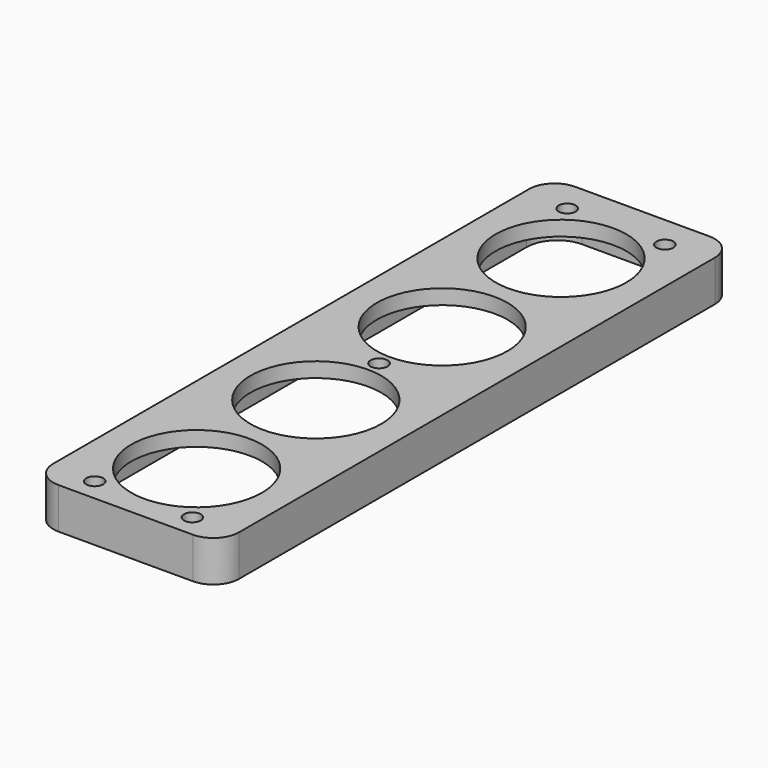
from build123d import *

# Parameters (mm, degrees)
F1_START      = 3.1
F0_W          = 32
F0_H          = 122
F0_R          = 1.65
F0_R_2        = 1.25
F0_R_3        = 12.75
F1_DEPTH      = 2.9
F2_START      = 3
F0_R_4        = 2
F0_R_5        = 1
F2_DEPTH      = 2
F3_DEPTH      = 25
F3_DEPTH_BACK = 39.8
F0_W_2        = 36.2426135689
F0_H_2        = 125.9943731129
F4_DEPTH      = 2
F4_DEPTH_BACK = 6
F5_R          = 6
F6_R          = 5


# Not quite as in the source:
# - a feature names something its author has since deleted; it is built from what else it names


with BuildPart() as f1:
    # F0 (on Top) → F1 (new body)
    with BuildSketch(Plane.XY.offset(F1_START)):
        with Locations((0, 0.9860133167)):
            Rectangle(F0_W, F0_H)
        with Locations((-9.525, -57.4329458177)):
            Circle(F0_R, mode=Mode.SUBTRACT)
        with Locations((-9.525, -30.4671674967)):
            Circle(F0_R_2, mode=Mode.SUBTRACT)
        with Locations((0, -44.4789328166)):
            Circle(F0_R_3, mode=Mode.SUBTRACT)
        with Locations((-9.525, 0)):
            Circle(F0_R_2, mode=Mode.SUBTRACT)
        with Locations((0, -15.4157546586)):
            Circle(F0_R_3, mode=Mode.SUBTRACT)
        Circle(F0_R, mode=Mode.SUBTRACT)
        with Locations((9.525, -57.4329458177)):
            Circle(F0_R, mode=Mode.SUBTRACT)
        with Locations((9.525, -30.4671674967)):
            Circle(F0_R_2, mode=Mode.SUBTRACT)
        with Locations((9.525, 0)):
            Circle(F0_R_2, mode=Mode.SUBTRACT)
        with Locations((-9.525, 29.1974432766)):
            Circle(F0_R_2, mode=Mode.SUBTRACT)
        with Locations((0, 15.3948861798)):
            Circle(F0_R_3, mode=Mode.SUBTRACT)
        with Locations((-9.525, 57.7905103564)):
            Circle(F0_R, mode=Mode.SUBTRACT)
        with Locations((0, 44.3624239764)):
            Circle(F0_R_3, mode=Mode.SUBTRACT)
        with Locations((9.525, 29.1974432766)):
            Circle(F0_R_2, mode=Mode.SUBTRACT)
        with Locations((9.525, 57.7905103564)):
            Circle(F0_R, mode=Mode.SUBTRACT)
        with Locations((9.525, 0)):
            Circle(F0_R_2)
        with Locations((-9.525, 0)):
            Circle(F0_R_2)
        with Locations((9.525, 29.1974432766)):
            Circle(F0_R_2)
        with Locations((-9.525, 29.1974432766)):
            Circle(F0_R_2)
        with Locations((9.525, -30.4671674967)):
            Circle(F0_R_2)
        with Locations((-9.525, -30.4671674967)):
            Circle(F0_R_2)
        with Locations((9.525, -57.4329458177)):
            Circle(F0_R)
        with Locations((-9.525, -57.4329458177)):
            Circle(F0_R)
        Circle(F0_R)
        with Locations((9.525, 57.7905103564)):
            Circle(F0_R)
        with Locations((-9.525, 57.7905103564)):
            Circle(F0_R)
    extrude(amount=F1_DEPTH)

    # F0 (on Top) → F2 (cut)
    with BuildSketch(Plane.XY.offset(F2_START)):
        with Locations((0, 44.3624239764)):
            Circle(F0_R_3)
        with Locations((-9.525, 44.3624239764)):
            Circle(F0_R_4, mode=Mode.SUBTRACT)
        with Locations((9.525, 44.3624239764)):
            Circle(F0_R_4, mode=Mode.SUBTRACT)
        with Locations((0, 15.3948861798)):
            Circle(F0_R_3)
        with Locations((-9.525, 15.3948861798)):
            Circle(F0_R_4, mode=Mode.SUBTRACT)
        with Locations((9.525, 15.3948861798)):
            Circle(F0_R_4, mode=Mode.SUBTRACT)
        with Locations((0, -15.4157546586)):
            Circle(F0_R_3)
        with Locations((-9.525, -15.4157546586)):
            Circle(F0_R_4, mode=Mode.SUBTRACT)
        with Locations((9.525, -15.4157546586)):
            Circle(F0_R_4, mode=Mode.SUBTRACT)
        with Locations((0, -44.4789328166)):
            Circle(F0_R_3)
        with Locations((-9.525, -44.4789328166)):
            Circle(F0_R_4, mode=Mode.SUBTRACT)
        with Locations((9.525, -44.4789328166)):
            Circle(F0_R_4, mode=Mode.SUBTRACT)
        with Locations((9.525, 44.3624239764)):
            Circle(F0_R_4)
        with Locations((9.525, 44.3624239764)):
            Circle(F0_R_5, mode=Mode.SUBTRACT)
        with Locations((-9.525, 44.3624239764)):
            Circle(F0_R_4)
        with Locations((-9.525, 44.3624239764)):
            Circle(F0_R_5, mode=Mode.SUBTRACT)
        with Locations((9.525, 15.3948861798)):
            Circle(F0_R_4)
        with Locations((9.525, 15.3948861798)):
            Circle(F0_R_5, mode=Mode.SUBTRACT)
        with Locations((-9.525, 15.3948861798)):
            Circle(F0_R_4)
        with Locations((-9.525, 15.3948861798)):
            Circle(F0_R_5, mode=Mode.SUBTRACT)
        with Locations((9.525, -15.4157546586)):
            Circle(F0_R_4)
        with Locations((9.525, -15.4157546586)):
            Circle(F0_R_5, mode=Mode.SUBTRACT)
        with Locations((-9.525, -15.4157546586)):
            Circle(F0_R_4)
        with Locations((-9.525, -15.4157546586)):
            Circle(F0_R_5, mode=Mode.SUBTRACT)
        with Locations((9.525, -44.4789328166)):
            Circle(F0_R_4)
        with Locations((9.525, -44.4789328166)):
            Circle(F0_R_5, mode=Mode.SUBTRACT)
        with Locations((-9.525, -44.4789328166)):
            Circle(F0_R_4)
        with Locations((-9.525, -44.4789328166)):
            Circle(F0_R_5, mode=Mode.SUBTRACT)
        with Locations((9.525, 44.3624239764)):
            Circle(F0_R_5)
        with Locations((-9.525, 44.3624239764)):
            Circle(F0_R_5)
        with Locations((9.525, 15.3948861798)):
            Circle(F0_R_5)
        with Locations((-9.525, 15.3948861798)):
            Circle(F0_R_5)
        with Locations((9.525, -15.4157546586)):
            Circle(F0_R_5)
        with Locations((-9.525, -15.4157546586)):
            Circle(F0_R_5)
        with Locations((9.525, -44.4789328166)):
            Circle(F0_R_5)
        with Locations((-9.525, -44.4789328166)):
            Circle(F0_R_5)
    extrude(amount=F2_DEPTH, mode=Mode.SUBTRACT)

    # F0 (on Top) → F3 (cut, two sides)
    with BuildSketch(Plane.XY) as f3_sk:
        with Locations((9.525, -57.4329458177)):
            Circle(F0_R)
        Circle(F0_R)
        with Locations((-9.525, -57.4329458177)):
            Circle(F0_R)
        with Locations((-9.525, 57.7905103564)):
            Circle(F0_R)
        with Locations((9.525, 57.7905103564)):
            Circle(F0_R)
    extrude(amount=-F3_DEPTH, mode=Mode.SUBTRACT)
    extrude(f3_sk.sketch, amount=F3_DEPTH_BACK, mode=Mode.SUBTRACT)

    # F0 (on Top) → F4 (join, two sides)
    with BuildSketch(Plane.XY) as f4_sk:
        with Locations((0.0427393243, 1.1539515108)):
            Rectangle(F0_W_2, F0_H_2)
        with Locations((0, 0.9860133167)):
            Rectangle(F0_W, F0_H, mode=Mode.SUBTRACT)
    extrude(amount=-F4_DEPTH)
    extrude(f4_sk.sketch, amount=F4_DEPTH_BACK)

    # F5
    f5_edges = [f1.edges().sort_by_distance(p)[0] for p in [
        (-16, -60.013987, 0.55),
        (16, -60.013987, 0.55),
        (-16, 61.986013, 0.55),
        (16, 61.986013, 0.55),
    ]]
    fillet(f5_edges, radius=F5_R)

    # F6
    f6_edges = [f1.edges().sort_by_distance(p)[0] for p in [
        (18.164046, 64.151138, 2),
        (-18.078567, 64.151138, 2),
        (-18.078567, -61.843235, 2),
        (18.164046, -61.843235, 2),
    ]]
    fillet(f6_edges, radius=F6_R)


solid = f1.part
